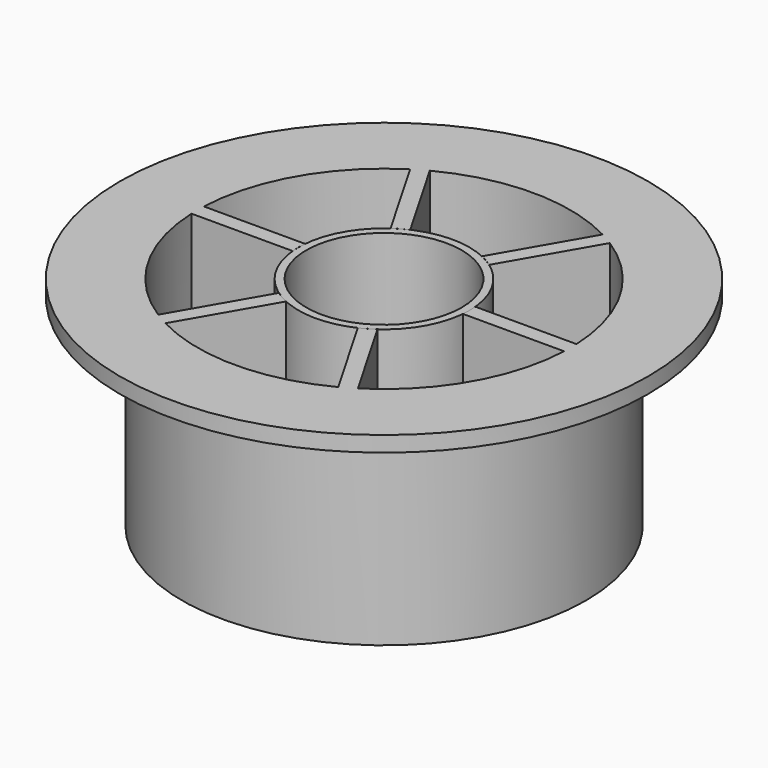
from build123d import *

# Parameters (mm, degrees)
F2_R     = 11
F2_R_2   = 10
F3_DEPTH = 28
F5_DEPTH = 28


with BuildPart() as f1:
    # F0 (on Front) → F1 (revolve)
    with BuildSketch(Plane.XZ):
        Polygon((34, 0), (24, 0), (24, -28), (26, -28), (26, -2), (34, -2), align=None)
    revolve(axis=Axis((0, 0, -3.8373200223), (0, 0, -1)))

    # F4 (on face) → F5 (join, through all)
    with BuildSketch(Plane(origin=(0, 0, -28), x_dir=(1, 0, 0), z_dir=(0, 0, -1))):
        with BuildLine():
            Line((-10.9544511501, 1), (-23.9791576166, 1))
            ThreePointArc((-23.9791576166, 1), (-24, 0), (-23.9791576166, -1))
            Line((-23.9791576166, -1), (-10.9544511501, -1))
            ThreePointArc((-10.9544511501, -1), (-11, 0), (-10.9544511501, 1))
        make_face()
        with BuildLine():
            Line((-6.3432509788, -8.9868329805), (-12.8556042121, -20.2665596573))
            ThreePointArc((-12.8556042121, -20.2665596573), (-12, -20.7846096908), (-11.1235534045, -21.2665596573))
            Line((-11.1235534045, -21.2665596573), (-4.6112001713, -9.9868329805))
            ThreePointArc((-4.6112001713, -9.9868329805), (-5.5, -9.5262794416), (-6.3432509788, -8.9868329805))
        make_face()
        with BuildLine():
            Line((4.6112001713, -9.9868329805), (11.1235534045, -21.2665596573))
            ThreePointArc((11.1235534045, -21.2665596573), (12, -20.7846096908), (12.8556042121, -20.2665596573))
            Line((12.8556042121, -20.2665596573), (6.3432509788, -8.9868329805))
            ThreePointArc((6.3432509788, -8.9868329805), (5.5, -9.5262794416), (4.6112001713, -9.9868329805))
        make_face()
        with BuildLine():
            Line((10.9544511501, -1), (23.9791576166, -1))
            ThreePointArc((23.9791576166, -1), (24, 0), (23.9791576166, 1))
            Line((23.9791576166, 1), (10.9544511501, 1))
            ThreePointArc((10.9544511501, 1), (11, 0), (10.9544511501, -1))
        make_face()
        with BuildLine():
            Line((6.3432509788, 8.9868329805), (12.8556042121, 20.2665596573))
            ThreePointArc((12.8556042121, 20.2665596573), (12, 20.7846096908), (11.1235534045, 21.2665596573))
            Line((11.1235534045, 21.2665596573), (4.6112001713, 9.9868329805))
            ThreePointArc((4.6112001713, 9.9868329805), (5.5, 9.5262794416), (6.3432509788, 8.9868329805))
        make_face()
        with BuildLine():
            Line((-4.6112001713, 9.9868329805), (-11.1235534045, 21.2665596573))
            ThreePointArc((-11.1235534045, 21.2665596573), (-12, 20.7846096908), (-12.8556042121, 20.2665596573))
            Line((-12.8556042121, 20.2665596573), (-6.3432509788, 8.9868329805))
            ThreePointArc((-6.3432509788, 8.9868329805), (-5.5, 9.5262794416), (-4.6112001713, 9.9868329805))
        make_face()
    extrude(amount=-F5_DEPTH)


with BuildPart() as f3:
    # F2 (on Top) → F3 (new body, through all)
    with BuildSketch(Plane.XY):
        Circle(F2_R)
        Circle(F2_R_2, mode=Mode.SUBTRACT)
    extrude(amount=-F3_DEPTH)


solid = Compound([f1.part, f3.part])
